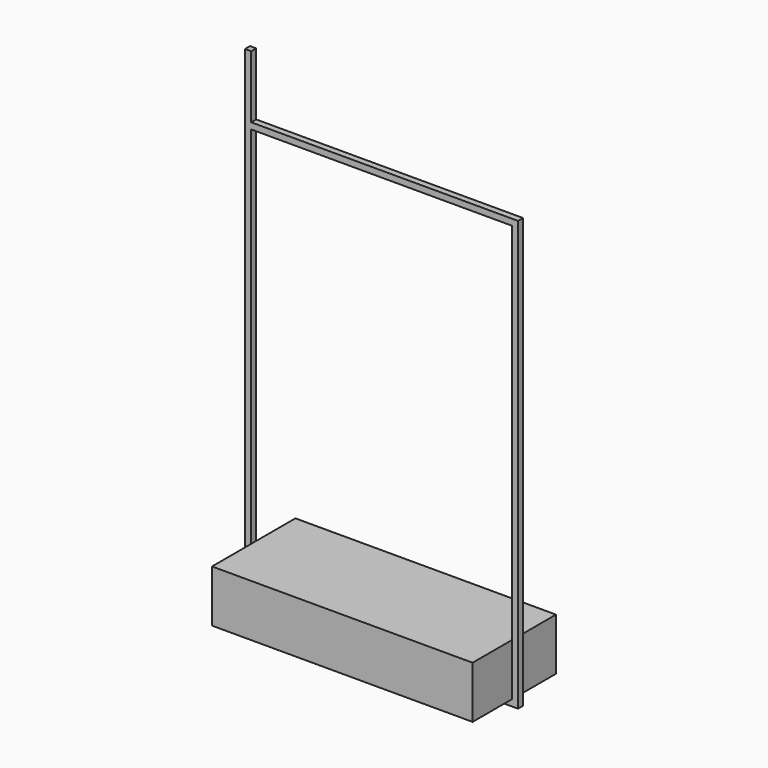
from build123d import *

# Parameters (mm, degrees)
F0_W     = 1250
F0_H     = 500
F1_DEPTH = 250
F2_W     = 1310
F2_H     = 2060
F2_W_2   = 1250
F2_H_2   = 2000
F3_DEPTH = 15
F4_W     = 1050
F4_H     = 300
F4_W_2   = 990
F4_H_2   = 240
F5_DEPTH = 30
F6_W     = 30
F6_H     = 30
F7_DEPTH = 300


with BuildPart() as f1:
    # F0 (on Top) → F1 (new body)
    with BuildSketch(Plane.XY):
        Rectangle(F0_W, F0_H)
    extrude(amount=F1_DEPTH)


with BuildPart() as f3:
    # F2 (on Front) → F3 (new body, symmetric)
    with BuildSketch(Plane.XZ):
        with Locations((0, 1000)):
            Rectangle(F2_W, F2_H)
        with Locations((0, 1000)):
            Rectangle(F2_W_2, F2_H_2, mode=Mode.SUBTRACT)
    extrude(amount=F3_DEPTH, both=True)

    # F4 (on face) → F5 (join)
    with BuildSketch(Plane(origin=(0, 0, 0), x_dir=(1, 0, 0), z_dir=(0, 0, -1))):
        Rectangle(F4_W, F4_H)
        Rectangle(F4_W_2, F4_H_2, mode=Mode.SUBTRACT)
    extrude(amount=F5_DEPTH)

    # F6 (on face) → F7 (join)
    with BuildSketch(Plane.XY.offset(2030)):
        with Locations((-640, 0)):
            Rectangle(F6_W, F6_H)
    extrude(amount=F7_DEPTH)


solid = Compound([f1.part, f3.part])
